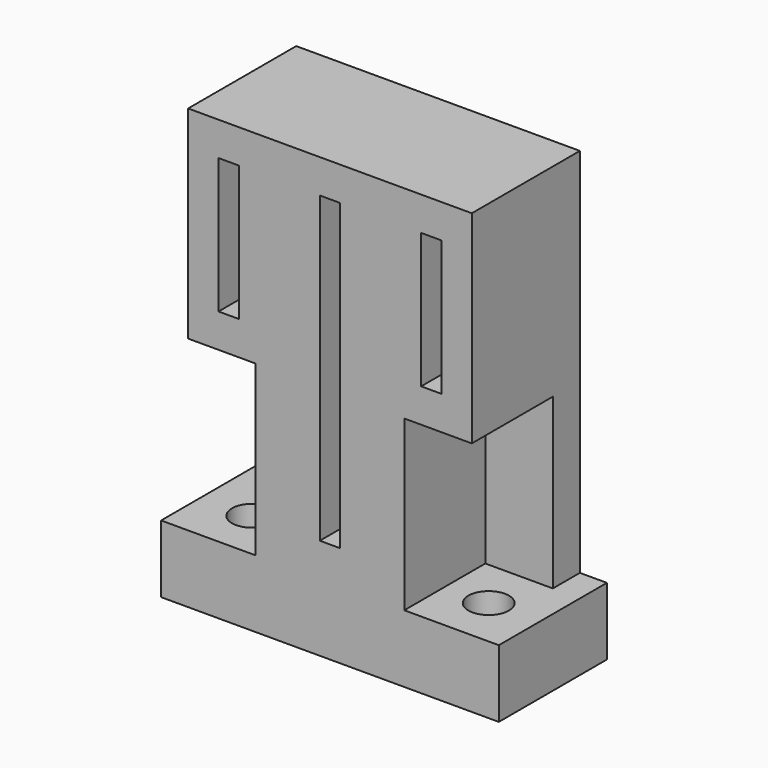
from build123d import *

# Parameters (mm, degrees)
F0_W     = 50
F0_H     = 20
F0_R     = 3
F1_DEPTH = 10
F2_W     = 42
F2_H     = 55
F3_DEPTH = 20
F4_W     = 3
F4_H     = 20
F4_H_2   = 45
F5_DEPTH = 20
F6_W     = 15
F6_H     = 25
F7_DEPTH = 10


# Not quite as in the source:
# - a pattern or mirror of a feature is missing from the dataset's text; its kind, count and spacing are read off the source's solid


with BuildPart() as f1:
    # F0 (on Top) → F1 (new body)
    with BuildSketch(Plane.XY):
        with Locations((0, -2.5)):
            Rectangle(F0_W, F0_H)
        with Locations((-17.5, -5)):
            Circle(F0_R, mode=Mode.SUBTRACT)
        with Locations((17.5, -5)):
            Circle(F0_R, mode=Mode.SUBTRACT)
    extrude(amount=F1_DEPTH)

    # F2 (on face) → F3 (join)
    with BuildSketch(Plane(origin=(0, 7.5, 0), x_dir=(-1, 0, 0), z_dir=(0, 1, 0))):
        with Locations((0, 37.5)):
            Rectangle(F2_W, F2_H)
    extrude(amount=-F3_DEPTH)

    # F4 (on face) → F5 (cut, through all)
    with BuildSketch(Plane(origin=(0, 7.5, 0), x_dir=(-1, 0, 0), z_dir=(0, 1, 0))):
        with Locations((-15, 50)):
            Rectangle(F4_W, F4_H)
        with Locations((0, 37.5)):
            Rectangle(F4_W, F4_H_2)
        with Locations((15, 50)):
            Rectangle(F4_W, F4_H)
    extrude(amount=-F5_DEPTH, mode=Mode.SUBTRACT)

    # F6 (on face) → F7 (cut)
    with BuildSketch(Plane.YZ.offset(21)):
        with Locations((-5, 22.5)):
            Rectangle(F6_W, F6_H)
    f7 = extrude(amount=-F7_DEPTH, mode=Mode.SUBTRACT)

    # F7_copies: F7 across plane
    add(f7.mirror(Plane(origin=(0, 0, 0), x_dir=(0, 0, -1), z_dir=(-1, 0, 0))), mode=Mode.SUBTRACT)


solid = f1.part
